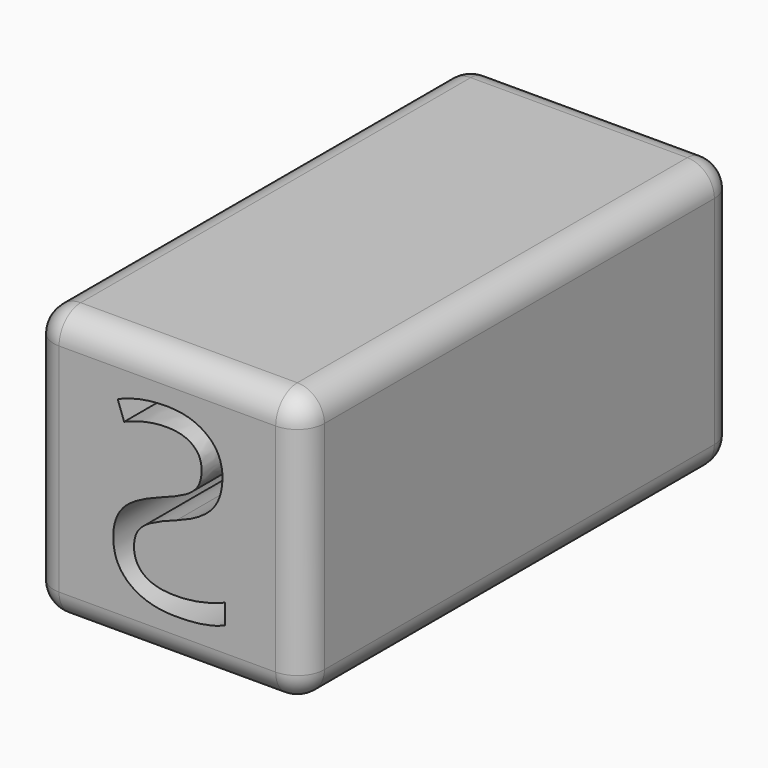
from build123d import *

# Parameters (mm, degrees)
F0_W         = 10
F0_H         = 10
F1_DEPTH     = 20
F2_R         = 1
F3_TEXT_SIZE = 9.1666666667
F4_DEPTH     = 25


# Not quite as in the source:
# - Text() gives the source's letters only with a copy of the font that has no kerning and outlines rounded to 1/6400 em; it was checked with that copy


with BuildPart() as f1:
    # F0 (on Front) → F1 (new body)
    with BuildSketch(Plane.XZ):
        with Locations((5, 5)):
            Rectangle(F0_W, F0_H)
    extrude(amount=F1_DEPTH)

    # F2
    f2_edges = [f1.edges().sort_by_distance(p)[0] for p in [
        (10, -10, 10),
        (0, -10, 10),
        (5, 0, 10),
        (5, -20, 10),
        (10, -10, 0),
        (10, 0, 5),
        (10, -20, 5),
        (0, -10, 0),
        (5, 0, 0),
        (5, -20, 0),
        (0, 0, 5),
        (0, -20, 5),
    ]]
    fillet(f2_edges, radius=F2_R)

    # F3 (on face) → F4 (cut)
    with BuildSketch(Plane(origin=(0, 0, 0), x_dir=(-1, 0, 0), z_dir=(0, 1, 0))):
        with Locations((-7.5931640625, 1.7)):
            Text('S', F3_TEXT_SIZE, font='Open Sans', text_align=(TextAlign.LEFT, TextAlign.BOTTOM))
    extrude(amount=-F4_DEPTH, mode=Mode.SUBTRACT)


solid = f1.part
